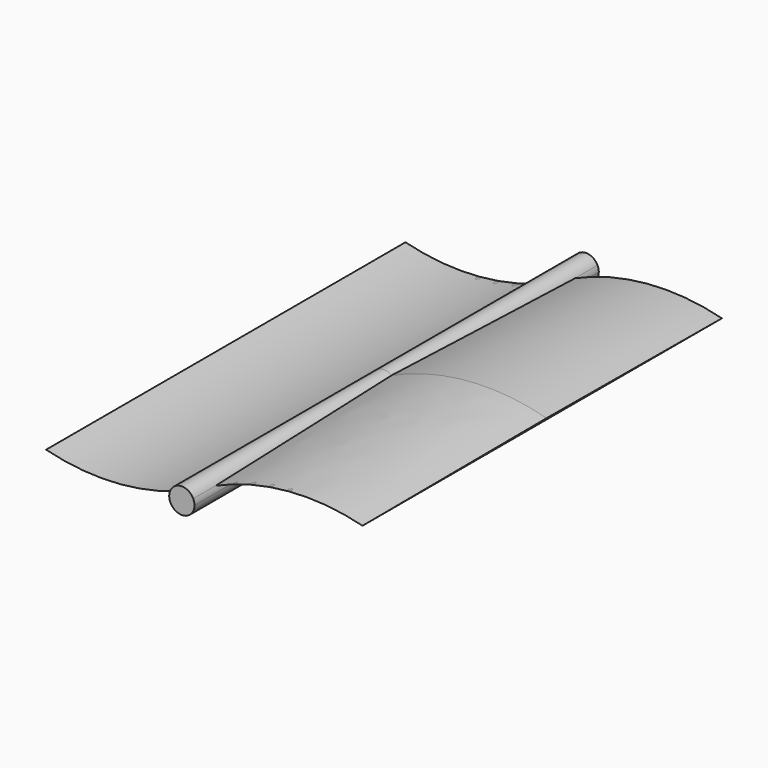
from build123d import *

# Parameters (mm, degrees)
F4_DEPTH = 360


with BuildPart() as f2:
    # F2: sweep along a path in F0
    with BuildLine(Plane.XZ) as f2_path:
        ThreePointArc((242.7527745604, 20.7435647383), (128.2776322592, 35.2070479661), (16.1666904568, 7.9144247848))
    # F1 (on Right) → F2 (sweep)
    with BuildSketch(Plane.YZ):
        Polygon((-320, 0), (0, 0), (320, 0), (0, 9.1953519732), align=None)
    sweep(path=f2_path.line)

    # F3: sweep along a path in F0
    with BuildLine(Plane.XZ) as f3_path:
        ThreePointArc((-242.7527745604, -20.7435647383), (-128.2776322592, -35.2070479661), (-16.1666904568, -7.9144247848))
    # F1 (on Right) → F3 (sweep)
    with BuildSketch(Plane.YZ):
        Polygon((320, 0), (0, 0), (-320, 0), (0, -9.1953519732), align=None)
    sweep(path=f3_path.line)

    # F0 (on Front) → F4 (join, symmetric)
    with BuildSketch(Plane.XZ):
        with BuildLine():
            ThreePointArc((-16.1666904568, -7.9144247848), (4.061992847, -17.5356840218), (18, 0))
            ThreePointArc((18, 0), (17.5356840218, 4.061992847), (16.1666904568, 7.9144247848))
            ThreePointArc((16.1666904568, 7.9144247848), (-7.9144247848, 16.1666904568), (-16.1666904568, -7.9144247848))
        make_face()
    extrude(amount=F4_DEPTH, both=True)


solid = f2.part
